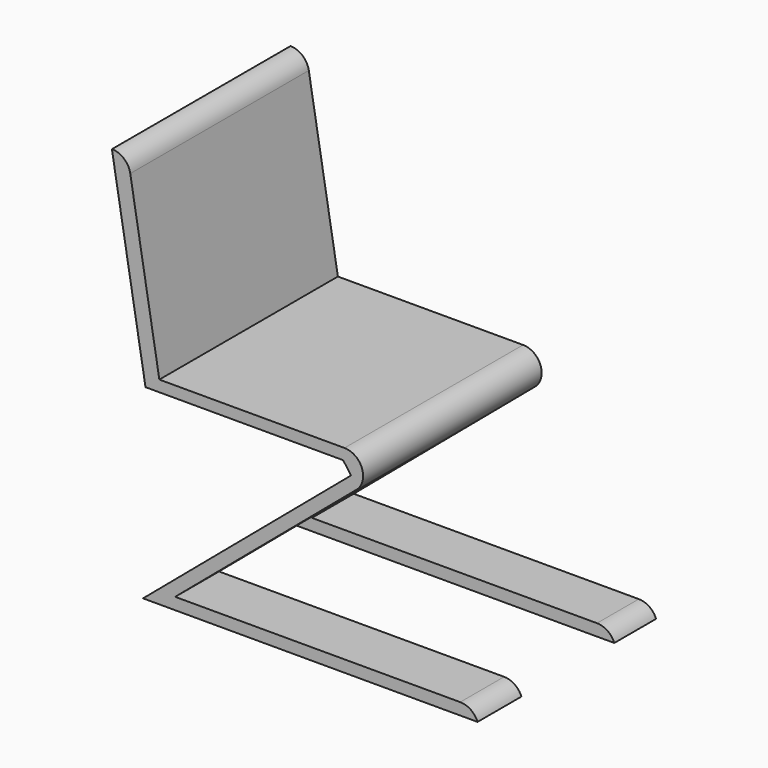
from build123d import *

# Parameters (mm, degrees)
F1_DEPTH      = 60
F2_T1_DEPTH   = 128.3050587773
F2_T3_DEPTH   = 87.2325127198
F2_T5_DEPTH   = 83.2679866238
F3_W          = 31.2075465918
F3_H          = 53.4305032343
F4_DEPTH      = 47.1568533609
F4_DEPTH_BACK = 100


# Not quite as in the source:
# - a fillet or chamfer that OpenCascade refuses, or shapes differently, is made with other operations: its cross-section is extruded or revolved along the edge and cut away or added


with BuildPart() as f1:
    # F0 (on Front) → F1 (new body)
    with BuildSketch(Plane.XZ):
        Polygon((-43.1315037153, 54.6031631236), (-47.1558533609, 53.3990226686), (-38.1231829524, 0), (15.0101743639, 0), (17.1355064958, -2.9223344754), (-27.4965111166, -40.6470149755), (-38.7919515192, -50.1943512397), (51.1408522725, -50.1943512397), (51.1408522725, -47.0230206847), (-30.1531795412, -47.0230206847), (19.4947316054, -5.0587160063), (29.0376522148, 3.0073238074), (-34.4038493931, 3.0073238074), align=None)
    extrude(amount=F1_DEPTH)

    # F2: fillet of radius 5 on 3 edges, made by hand

    # F2_s2 → F2_t1 (cut)
    with BuildSketch(Plane.XZ.offset(-34.1525293886)):
        with BuildLine():
            ThreePointArc((18.6043132835, -5.8113314716), (20.0720252356, -0.274141409), (15.3766404593, 3.0073238074))
            Line((15.3766404593, 3.0073238074), (29.0376522148, 3.0073238074))
            Line((29.0376522148, 3.0073238074), (18.6043132835, -5.8113314716))
        make_face()
    extrude(amount=F2_T1_DEPTH, mode=Mode.SUBTRACT)

    # F2_s4 → F2_t3 (cut)
    with BuildSketch(Plane.XZ.offset(-13.6162563599)):
        with BuildLine():
            ThreePointArc((-47.1558533609, 53.3990226686), (-43.9268794892, 52.21892637), (-42.2231091456, 49.2329481124))
            Line((-42.2231091456, 49.2329481124), (-43.1315037153, 54.6031631236))
            Line((-43.1315037153, 54.6031631236), (-47.1558533609, 53.3990226686))
        make_face()
    extrude(amount=F2_T3_DEPTH, mode=Mode.SUBTRACT)

    # F2_s6 → F2_t5 (cut)
    with BuildSketch(Plane.XZ.offset(-11.6339933119)):
        with BuildLine():
            ThreePointArc((51.1408522725, -50.1943512397), (49.3029833415, -47.8912324989), (46.4872549478, -47.0230206847))
            Line((46.4872549478, -47.0230206847), (51.1408522725, -47.0230206847))
            Line((51.1408522725, -47.0230206847), (51.1408522725, -50.1943512397))
        make_face()
    extrude(amount=F2_T5_DEPTH, mode=Mode.SUBTRACT)

    # F3 (on Right) → F4 (cut, two sides)
    with BuildSketch(Plane.YZ) as f4_sk:
        with Locations((-29.6471677721, -47.0001557842)):
            Rectangle(F3_W, F3_H)
    extrude(amount=-F4_DEPTH, mode=Mode.SUBTRACT)
    extrude(f4_sk.sketch, amount=F4_DEPTH_BACK, mode=Mode.SUBTRACT)


solid = f1.part
